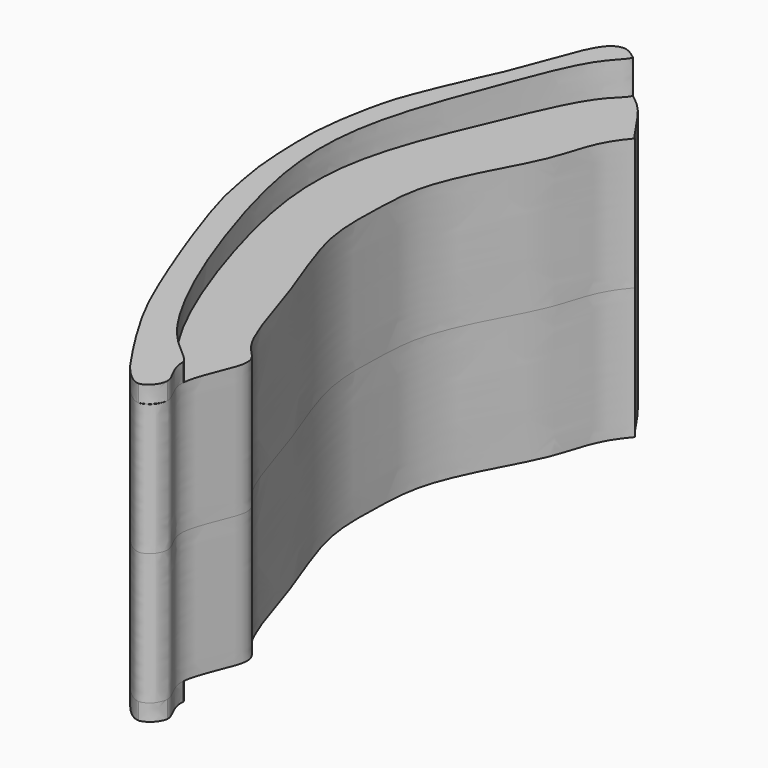
from build123d import *

# Parameters (mm, degrees)
F1_DEPTH      = 9.3091
F3_DEPTH      = 2.54
F3_DEPTH_BACK = 21.1582
F5_DEPTH      = 25.4


with BuildPart() as f1:
    # F0 (on Top) → F1 (new body, symmetric)
    with BuildSketch(Plane.XY):
        with BuildLine():
            add(Edge.make_bspline(
                [(-4.6924524078, 0), (-5.4936572119, -0.2330396403), (-6.8452489509, -3.4171227576), (-7.9782609963, -6.3294147105), (-9.3798685225, -8.7562191453), (-10.8811095897, -12.1083774015), (-11.7885979825, -15.8081023922), (-12.1804042879, -19.2229627562), (-12.0834048314, -22.3589626101), (-11.4618145886, -26.2871085681), (-10.7298705876, -29.3462376356), (-8.900462661, -34.1745497485), (-6.7928083907, -39.7227092724), (-4.2693992015, -43.8383388891), (-1.8164845814, -47.0008237268), (-0.843006876, -45.8786030837), (-0.8436239212, -45.8794316554), (-0.1762218328, -44.8883165662), (-2.1562975675, -43.1823030814), (0.8121486303, -38.5493219827), (-1.3282871319, -37.4142446948), (-2.7596097616, -32.9141990314), (-3.9590141984, -29.2535049739), (-6.0096731064, -24.2620182586), (-5.8529272193, -20.086819125), (-5.781222482, -16.3868914166), (-3.6890598085, -12.075157629), (-1.9835534282, -9.0706185099), (-1.3363463278, -5.9747729629), (0.0644609254, -4.4126354132), (-0.0959687699, -4.5405297218), (-1.8347783472, -1.6879475745), (-2.9332250938, -0.8370678411), (-4.147579909, 0.1584824386), (-4.6924524078, 0)],
                knots=[0, 0, 0, 0, 0.0357607937, 0.0698190244, 0.1000505632, 0.1351596078, 0.1712640858, 0.2050435863, 0.2377519071, 0.2739325598, 0.3066375111, 0.3481151164, 0.3931915502, 0.4352958211, 0.4683344634, 0.4851514983, 0.4869046803, 0.5032901746, 0.5301211862, 0.569100922, 0.5937971845, 0.6326802218, 0.6701292011, 0.7122293877, 0.7495610901, 0.7847247206, 0.8245082169, 0.8589531515, 0.8928139704, 0.9160804057, 0.9186872058, 0.9503860572, 0.9756802844, 1, 1, 1, 1], degree=3))
        make_face()
    extrude(amount=F1_DEPTH, both=True)

    # F2 (on face) → F3 (join, two sides)
    with BuildSketch(Plane.XY.offset(9.3091)) as f3_sk:
        with BuildLine():
            add(Edge.make_bspline(
                [(-3.2921972659, -0.539879962), (-3.3223764028, -0.8388564779), (-4.9069759769, -2.0229615857), (-7.1203679307, -7.3190732948), (-10.4333900863, -14.8603156066), (-10.8789268102, -21.8614251752), (-8.6463054538, -29.9693054682), (-6.3114725318, -36.2406411391), (-3.5274172579, -41.1499875419), (-1.4835509623, -42.3838091982), (-1.2359984666, -42.8872194769)],
                knots=[0.002652301, 0.002652301, 0.002652301, 0.002652301, 0.0287439733, 0.0828381309, 0.1468375981, 0.2052014192, 0.2688498826, 0.3271258172, 0.3794673737, 0.4148550205, 0.4148550205, 0.4148550205, 0.4148550205], degree=3))
            add(Edge.make_bspline(
                [(-3.2921972589, -0.5398799603), (-3.5828646883, -0.3117827132), (-3.909366051, -0.0813464674), (-4.2356584124, 0)],
                knots=[0.9791191631, 0.9791191631, 0.9791191631, 0.9791191631, 0.9933177178, 0.9933177178, 0.9933177178, 0.9933177178], degree=3))
            add(Edge.make_bspline(
                [(-5.4050003361, -0.5690377681), (-5.0672274202, -0.1663065652), (-4.6896468707, 0.0218062498), (-4.2356584124, 0)],
                knots=[0.9521834174, 0.9521834174, 0.9521834174, 0.9521834174, 0.9774257296, 0.9774257296, 0.9774257296, 0.9774257296], degree=3))
            add(Edge.make_bspline(
                [(-5.4050003361, -0.5690377681), (-5.625753654, -0.8521769755), (-5.8354620449, -1.2149532857), (-6.0330683929, -1.6103555454)],
                knots=[0.0110853662, 0.0110853662, 0.0110853662, 0.0110853662, 0.021899521, 0.021899521, 0.021899521, 0.021899521], degree=3))
            add(Edge.make_bspline(
                [(-7.2536345734, -4.4743160077), (-6.77217415, -3.3668805455), (-6.4005135491, -2.3736916286), (-6.0330683929, -1.6103555454)],
                knots=[0.9061725015, 0.9061725015, 0.9061725015, 0.9061725015, 0.9357275898, 0.9357275898, 0.9357275898, 0.9357275898], degree=3))
            add(Edge.make_bspline(
                [(-7.2536345734, -4.4743160077), (-7.5375497973, -5.1683476962), (-7.9741480577, -6.2066239029), (-8.4692752193, -7.1459615397), (-8.6791956284, -7.5393337525)],
                knots=[0.0481543081, 0.0481543081, 0.0481543081, 0.0481543081, 0.0698190244, 0.0849681337, 0.0849681337, 0.0849681337, 0.0849681337], degree=3))
            add(Edge.make_bspline(
                [(-10.7777390643, -12.1656069887), (-10.2327790902, -10.7666680312), (-9.4470947797, -9.1393502327), (-8.6791956284, -7.5393337525)],
                knots=[0.8417891742, 0.8417891742, 0.8417891742, 0.8417891742, 0.880541255, 0.880541255, 0.880541255, 0.880541255], degree=3))
            add(Edge.make_bspline(
                [(-10.7777390643, -12.1656069887), (-11.1933522731, -13.3814203517), (-11.6620975085, -15.2994690211), (-11.9261488346, -17.1346907064), (-11.9925246347, -17.7576877529)],
                knots=[0.1356687779, 0.1356687779, 0.1356687779, 0.1356687779, 0.1712640858, 0.1901222963, 0.1901222963, 0.1901222963, 0.1901222963], degree=3))
            add(Edge.make_bspline(
                [(-11.9614663037, -22.8020705624), (-12.0892154847, -21.2044393231), (-12.1033725955, -19.3919632569), (-11.9925246347, -17.7576877529)],
                knots=[0.739103964, 0.739103964, 0.739103964, 0.739103964, 0.7854496122, 0.7854496122, 0.7854496122, 0.7854496122], degree=3))
            add(Edge.make_bspline(
                [(-11.9614663037, -22.8020705624), (-11.8336241356, -23.9340777879), (-11.6123388066, -25.3024743428), (-11.3813932676, -26.4650447138), (-11.3563375975, -26.5878609344)],
                knots=[0.2418000813, 0.2418000813, 0.2418000813, 0.2418000813, 0.2739325598, 0.2777897931, 0.2777897931, 0.2777897931, 0.2777897931], degree=3))
            add(Edge.make_bspline(
                [(-8.5896455976, -34.9892573056), (-9.406586429, -32.8407548702), (-10.5799595621, -29.5189543), (-11.2370855686, -27.07978453), (-11.3563375975, -26.5878609344)],
                knots=[0.6353661476, 0.6353661476, 0.6353661476, 0.6353661476, 0.6874509886, 0.7014059726, 0.7014059726, 0.7014059726, 0.7014059726], degree=3))
            add(Edge.make_bspline(
                [(-8.5896455976, -34.9892573056), (-8.380566356, -35.5365098634), (-8.1683386322, -36.0853313913), (-7.9509643964, -36.6292398124)],
                knots=[0.3553353616, 0.3553353616, 0.3553353616, 0.3553353616, 0.3683538436, 0.3683538436, 0.3683538436, 0.3683538436], degree=3))
            add(Edge.make_bspline(
                [(-3.3456171826, -44.9696762451), (-3.451295436, -44.8204507822), (-4.4488880744, -43.3615102896), (-6.3702925924, -40.2929336574), (-7.3230161481, -38.1994751774), (-7.9509643964, -36.6292398124)],
                knots=[0.521525091, 0.521525091, 0.521525091, 0.521525091, 0.5273157546, 0.5759814304, 0.6210846781, 0.6210846781, 0.6210846781, 0.6210846781], degree=3))
            add(Edge.make_bspline(
                [(-3.3456171826, -44.9696762451), (-2.7698734567, -45.71094229), (-2.1842129963, -46.3057236046), (-1.6751513792, -46.3339385537)],
                knots=[0.4434066144, 0.4434066144, 0.4434066144, 0.4434066144, 0.4664925611, 0.4664925611, 0.4664925611, 0.4664925611], degree=3))
            add(Edge.make_bspline(
                [(-0.5735277076, -45.1495183647), (-0.6184665752, -45.6793796766), (-1.1546532309, -46.2906347834), (-1.6751513792, -46.3339385537)],
                knots=[0.4627907895, 0.4627907895, 0.4627907895, 0.4627907895, 0.4909428236, 0.4909428236, 0.4909428236, 0.4909428236], degree=3))
            add(Edge.make_bspline(
                [(-0.5735277076, -45.1495183647), (-0.573275788, -45.1418475467), (-0.5623729155, -44.5556126485), (-1.2677716796, -43.9478481158), (-1.2413084255, -42.9605181149), (-1.2359984666, -42.8872194769)],
                knots=[0.5029344549, 0.5029344549, 0.5029344549, 0.5029344549, 0.5032901746, 0.5301211862, 0.5322167325, 0.5322167325, 0.5322167325, 0.5322167325], degree=3))
        make_face()
    extrude(amount=F3_DEPTH)
    extrude(f3_sk.sketch, amount=-F3_DEPTH_BACK)

    # F4 (on Right) → F5 (cut)
    with BuildSketch(Plane.YZ):
        Polygon((-46.4445720829, 12.3205657469), (-46.4445720829, 10.5029), (2.9827478193, 11.7856), (2.9688647974, 12.3205657469), align=None)
        Polygon((-46.4445720829, -12.3205657469), (2.9688647974, -12.3205657469), (2.9827478193, -11.7856), (-46.4445720829, -10.5029), align=None)
    extrude(amount=-F5_DEPTH, mode=Mode.SUBTRACT)


solid = f1.part
